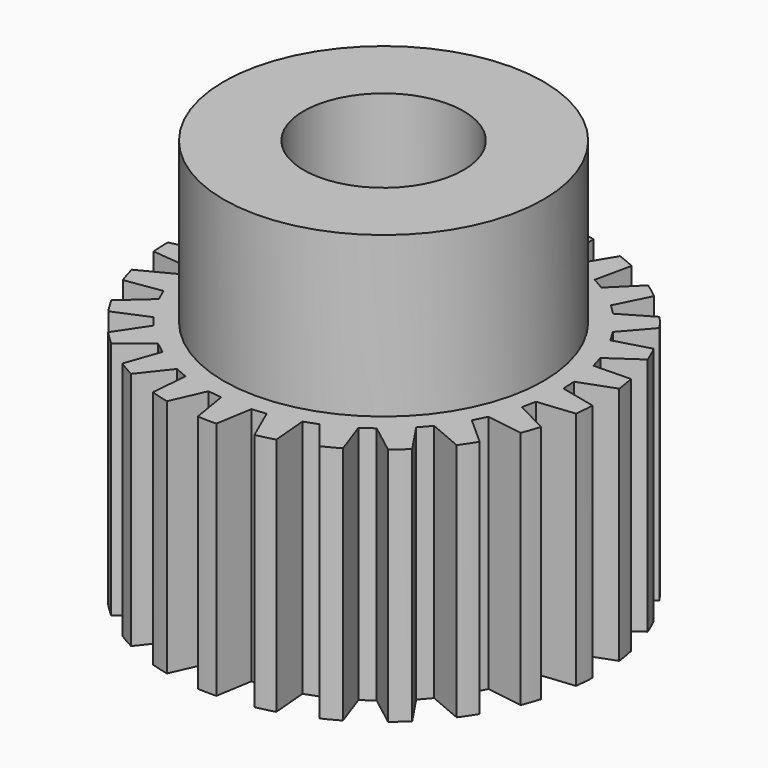
from build123d import *

# Parameters (mm, degrees)
F0_R            = 13.5
F1_DEPTH        = 15
F2_R            = 10
F3_DEPTH        = 10
F4_R            = 5
F5_DEPTH        = 25.001
F7_DEPTH        = 25.001
F7_COPIES_COUNT = 25


# Not quite as in the source:
# - a pattern or mirror of a feature is missing from the dataset's text; its kind, count and spacing are read off the source's solid


with BuildPart() as f1:
    # F0 (on Top) → F1 (new body)
    with BuildSketch(Plane.XY):
        Circle(F0_R)
    extrude(amount=F1_DEPTH)

    # F2 (on face) → F3 (join)
    with BuildSketch(Plane.XY.offset(15)):
        Circle(F2_R)
    extrude(amount=F3_DEPTH)

    # F4 (on face) → F5 (cut, through all)
    with BuildSketch(Plane.XY.offset(25)):
        Circle(F4_R)
    extrude(amount=-F5_DEPTH, mode=Mode.SUBTRACT)

    # F6 (on face) → F7 (cut, through all)
    with BuildSketch(Plane(origin=(0, 0, 0), x_dir=(1, 0, 0), z_dir=(0, 0, -1))):
        with BuildLine():
            Line((-13.3188989942, -2.2038442736), (-11.1612903898, -1.4099988776))
            Line((-11.1612903898, -1.4099988776), (-11.2378712938, -0.5222535625))
            Line((-11.2378712938, -0.5222535625), (-13.5, 0))
            ThreePointArc((-13.5, 0), (-13.4546485726, -1.1056363729), (-13.3188989942, -2.2038442736))
        make_face()
    f7 = extrude(amount=-F7_DEPTH, mode=Mode.SUBTRACT)

    # F7_copies: F7 ×25 about axis
    f7_copies_axis = Axis((0, 0, 0), (0, 0, 1))
    for i in range(1, F7_COPIES_COUNT):
        add(f7.rotate(f7_copies_axis, i * 360 / F7_COPIES_COUNT), mode=Mode.SUBTRACT)


solid = f1.part
